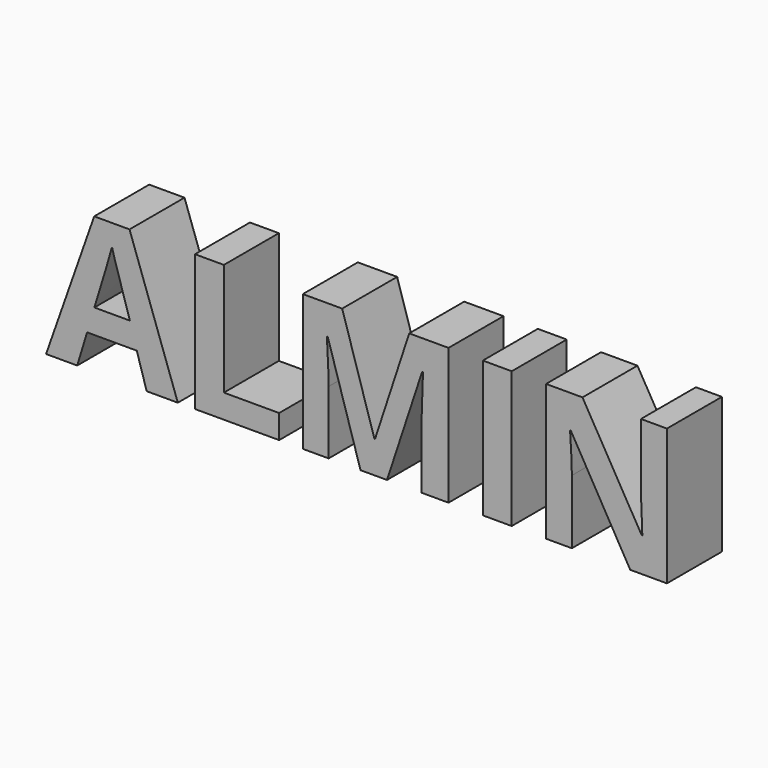
from build123d import *

# Parameters (mm, degrees)
F0_TEXT_SIZE = 69.4444444444
F1_DEPTH     = 25


# Not quite as in the source:
# - Text() gives the source's letters only with a copy of the font that has no kerning and outlines rounded to 1/6400 em; it was checked with that copy


with BuildPart() as f1:
    # F0 (on Front) → F1 (new body)
    with BuildSketch(Plane.XZ):
        with Locations((-97.1757345268, -15.8168472789)):
            Text('ALMIN', F0_TEXT_SIZE, font='Open Sans', font_style=FontStyle.BOLD, text_align=(TextAlign.LEFT, TextAlign.BOTTOM))
    extrude(amount=F1_DEPTH)


solid = f1.part
